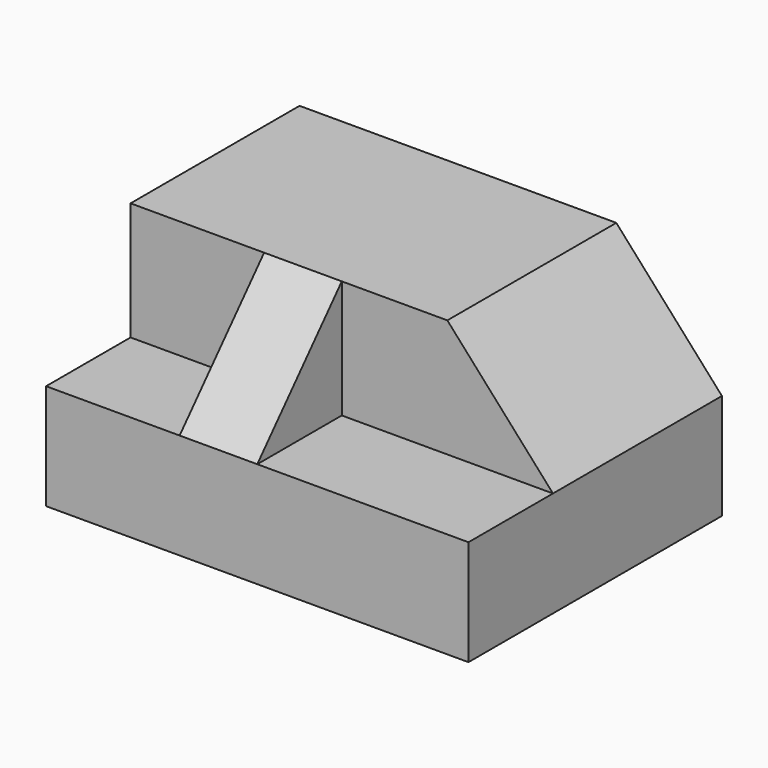
from build123d import *

# Parameters (mm, degrees)
F1_DEPTH = 25.4
F2_W     = 50.8
F2_H     = 12.7
F3_DEPTH = 12.7
F4_W     = 9.3365699251
F4_H     = 14.1990316571
F5_DEPTH = 12.7
F7_DEPTH = 25.4


# Not quite as in the source:
# - a feature names something its author has since deleted; it is built from what else it names


with BuildPart() as f1:
    # F0 (on Front) → F1 (new body)
    with BuildSketch(Plane.XZ):
        Polygon((-66.8362646442, 30.1552314789), (-66.8362646442, 3.2561998218), (-16.0362646442, 3.2561998218), (-16.0362646442, 15.9561998218), (-28.7362646442, 30.1552314789), align=None)
    extrude(amount=F1_DEPTH)

    # F2 (on face) → F3 (join)
    with BuildSketch(Plane.XZ.offset(25.4)):
        with Locations((-41.4362646442, 9.6061998218)):
            Rectangle(F2_W, F2_H)
    extrude(amount=F3_DEPTH)

    # F4 (on face) → F5 (join)
    with BuildSketch(Plane.XZ.offset(25.4)):
        with Locations((-46.1045496067, 23.0557156503)):
            Rectangle(F4_W, F4_H)
    extrude(amount=F5_DEPTH)

    # F6 (on face) → F7 (cut)
    with BuildSketch(Plane.YZ.offset(-41.4362646442)):
        Polygon((-38.1, 15.9561998218), (-25.4, 30.1552314789), (-38.1, 30.1552314789), align=None)
    extrude(amount=-F7_DEPTH, mode=Mode.SUBTRACT)


solid = f1.part
